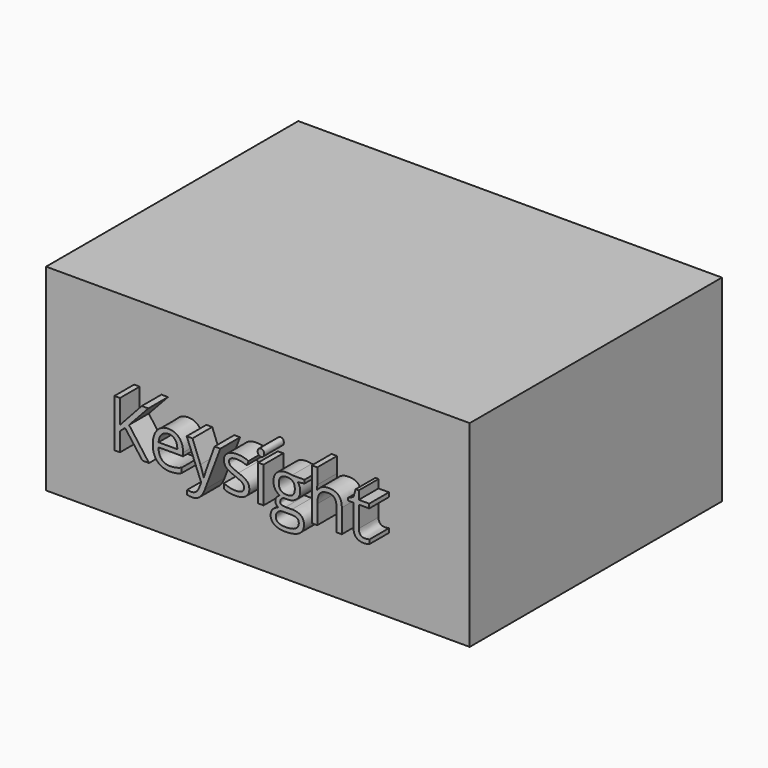
from build123d import *

# Parameters (mm, degrees)
F0_W         = 430
F0_H         = 200
F1_DEPTH     = 320
F2_TEXT_SIZE = 68.0481051354
F3_DEPTH     = 25


# Not quite as in the source:
# - Text() gives the source's letters only with a copy of the font that has no kerning and outlines rounded to 1/6400 em; it was checked with that copy


with BuildPart() as f1:
    # F0 (on Front) → F1 (new body)
    with BuildSketch(Plane.XZ):
        Rectangle(F0_W, F0_H)
    extrude(amount=F1_DEPTH)

    # F2 (on face) → F3 (join)
    with BuildSketch(Plane.XZ.offset(320)):
        with Locations((-132.2831269354, -24.8798984103)):
            Text('Keysight', F2_TEXT_SIZE, font='Open Sans', text_align=(TextAlign.LEFT, TextAlign.BOTTOM))
    extrude(amount=F3_DEPTH)


solid = f1.part
